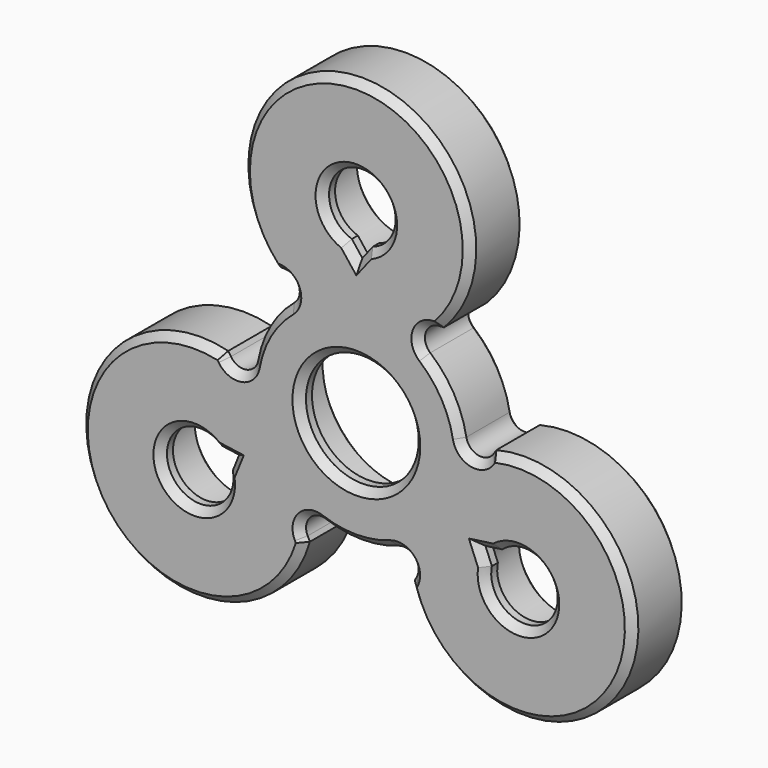
from build123d import *

# Parameters (mm, degrees)
F0_R        = 6.5
F0_R_2      = 11.05
F1_DEPTH    = 9.2
F2_R        = 7.5
F2_R_2      = 4.4268339864
F2_R_3      = 11.05
F3_DEPTH    = 2
F4_R        = 2
F6_DEPTH    = 25
F7_SIZE     = 1
F8_C1_SIZE  = 1
F8_C2_SIZE  = 1
F8_C3_SIZE  = 1
F8_C4_SIZE  = 1
F8_C5_SIZE  = 1
F8_C6_SIZE  = 1
F8_C7_SIZE  = 1
F8_C8_SIZE  = 1
F8_C9_SIZE  = 1
F8_C10_SIZE = 1
F8_C11_SIZE = 1
F8_C12_SIZE = 1
F8_C13_SIZE = 1
F8_C14_SIZE = 1
F8_C15_SIZE = 1
F8_C16_SIZE = 1


with BuildPart() as f1:
    # F0 (on Front) → F1 (new body)
    with BuildSketch(Plane.XZ):
        with BuildLine():
            Line((-10.8594483096, 14.3268800737), (-2.4829795671, 13.8288579597))
            ThreePointArc((-2.4829795671, 13.8288579597), (-12.1676569232, 7.025), (-13.217632082, -4.7641055977))
            Line((-13.217632082, -4.7641055977), (-17.8371662556, 2.2411180703))
            ThreePointArc((-17.8371662556, 2.2411180703), (-34.6870755728, -20.0265924193), (-6.977717946, -16.5679981441))
            Line((-6.977717946, -16.5679981441), (-10.7346525149, -9.064752362))
            ThreePointArc((-10.7346525149, -9.064752362), (0, -14.05), (10.7346525149, -9.064752362))
            Line((10.7346525149, -9.064752362), (6.977717946, -16.5679981441))
            ThreePointArc((6.977717946, -16.5679981441), (34.6870755728, -20.0265924193), (17.8371662556, 2.2411180703))
            Line((17.8371662556, 2.2411180703), (13.217632082, -4.7641055977))
            ThreePointArc((13.217632082, -4.7641055977), (12.1676569232, 7.025), (2.4829795671, 13.8288579597))
            Line((2.4829795671, 13.8288579597), (10.8594483096, 14.3268800737))
            ThreePointArc((10.8594483096, 14.3268800737), (0, 40.0531848387), (-10.8594483096, 14.3268800737))
        make_face()
        with Locations((-21.5623582929, -12.4490333648)):
            Circle(F0_R, mode=Mode.SUBTRACT)
        with Locations((21.5623582929, -12.4490333648)):
            Circle(F0_R, mode=Mode.SUBTRACT)
        Circle(F0_R_2, mode=Mode.SUBTRACT)
        with Locations((0, 24.8980667296)):
            Circle(F0_R, mode=Mode.SUBTRACT)
    extrude(amount=F1_DEPTH)

    # F2 (on face) → F3 (join)
    with BuildSketch(Plane.XZ.offset(9.2)):
        with Locations((0, 24.8980667296)):
            Circle(F2_R)
        with Locations((0, 24.8980667296)):
            Circle(F2_R_2, mode=Mode.SUBTRACT)
        with Locations((-21.5623582929, -12.4490333648)):
            Circle(F2_R)
        with Locations((-21.5623582929, -12.4490333648)):
            Circle(F2_R_2, mode=Mode.SUBTRACT)
        with Locations((21.5623582929, -12.4490333648)):
            Circle(F2_R)
        with Locations((21.5623582929, -12.4490333648)):
            Circle(F2_R_2, mode=Mode.SUBTRACT)
        Circle(F2_R_3)
        Circle(F2_R, mode=Mode.SUBTRACT)
    extrude(amount=-F3_DEPTH)

    # F4
    f4_edges = [f1.edges().sort_by_distance(p)[0] for p in [
        (2.48298, -4.6, 13.828858),
        (-2.48298, -4.6, 13.828858),
        (-13.217632, -4.6, -4.764106),
        (-10.734653, -4.6, -9.064752),
        (10.734653, -4.6, -9.064752),
        (13.217632, -4.6, -4.764106),
    ]]
    fillet(f4_edges, radius=F4_R)

    # F5 (on face) → F6 (cut)
    with BuildSketch(Plane.XZ.offset(9.2)):
        with BuildLine():
            Line((0, 18.9108662307), (1.7659365324, 21.1738422452))
            ThreePointArc((1.7659365324, 21.1738422452), (0, 24.9152206672), (-1.7659365324, 21.1738422452))
            Line((-1.7659365324, 21.1738422452), (0, 18.9108662307))
        make_face()
        with BuildLine():
            Line((-16.3772905634, -9.4554331154), (-19.2200535463, -9.057575224))
            ThreePointArc((-19.2200535463, -9.057575224), (-21.5772140387, -12.4576103336), (-17.4541170138, -12.1162670212))
            Line((-17.4541170138, -12.1162670212), (-16.3772905634, -9.4554331154))
        make_face()
        with BuildLine():
            Line((16.3772905634, -9.4554331154), (17.4541170138, -12.1162670212))
            ThreePointArc((17.4541170138, -12.1162670212), (21.5772140387, -12.4576103336), (19.2200535463, -9.057575224))
            Line((19.2200535463, -9.057575224), (16.3772905634, -9.4554331154))
        make_face()
    extrude(amount=-F6_DEPTH, mode=Mode.SUBTRACT)

    # F7
    f7_edges = [f1.edges().sort_by_distance(p)[0] for p in [
        (10.530932, 0, 14.307348),
        (8.422362, 0, 12.919623),
        (0, 0, 40.053185),
        (12.167657, 0, 7.025),
        (-10.530932, 0, 14.307348),
        (15.399903, 0, 0.834168),
        (-8.422362, 0, 12.919623),
        (17.655993, 0, 1.96638),
        (-12.167657, 0, 7.025),
        (34.687076, 0, -20.026592),
        (-15.399903, 0, 0.834168),
        (7.125061, 0, -16.273728),
        (-17.655993, 0, 1.96638),
        (6.977541, 0, -13.753791),
        (-34.687076, 0, -20.026592),
        (0, 0, -14.05),
        (-7.125061, 0, -16.273728),
        (-6.977541, 0, -13.753791),
        (-28.062358, 0, -12.449033),
        (15.062358, 0, -12.449033),
        (-11.05, 0, 0),
        (-6.5, 0, 24.898067),
    ]]
    chamfer(f7_edges, length=F7_SIZE)

    # F8: chamfer of 1 on 28 edges, made by hand

    # F8_c1
    f8_c1_edges = [f1.edges().sort_by_distance(p)[0] for p in [
        (10.5309316289, -9.2, 14.3073481472),
        (8.4223621743, -9.2, 12.9196228952),
        (17.6559927707, -9.2, 1.9663802425),
        (15.3999027217, -9.2, 0.8341681552),
        (12.1676569232, -9.2, 7.025),
    ]]
    chamfer(f8_c1_edges, length=F8_C1_SIZE)

    # F8_c2
    f8_c2_edges = [f1.edges().sort_by_distance(p)[0] for p in [
        (-10.5309316289, -9.2, 14.3073481472),
        (-8.4223621743, -9.2, 12.9196228952),
        (-12.1676569232, -9.2, 7.025),
        (-15.3999027217, -9.2, 0.8341681552),
        (-17.6559927707, -9.2, 1.9663802425),
    ]]
    chamfer(f8_c2_edges, length=F8_C2_SIZE)

    # F8_c3
    f8_c3_edges = [f1.edges().sort_by_distance(p)[0] for p in [
        (-7.1250611419, -9.2, -16.2737283897),
        (-6.9775405475, -9.2, -13.7537910504),
        (0, -9.2, -14.05),
        (6.9775405475, -9.2, -13.7537910504),
        (7.1250611419, -9.2, -16.2737283897),
    ]]
    chamfer(f8_c3_edges, length=F8_C3_SIZE)

    # F8_c4
    f8_c4_edges = [f1.edges().sort_by_distance(p)[0] for p in [
        (34.6870755728, -9.2, -20.0265924193),
    ]]
    chamfer(f8_c4_edges, length=F8_C4_SIZE)

    # F8_c5
    f8_c5_edges = [f1.edges().sort_by_distance(p)[0] for p in [
        (-25.3961089835, -9.2, -14.662450358),
    ]]
    chamfer(f8_c5_edges, length=F8_C5_SIZE)

    # F8_c6
    f8_c6_edges = [f1.edges().sort_by_distance(p)[0] for p in [
        (-16.7411021229, -9.2, -9.4045159968),
    ]]
    chamfer(f8_c6_edges, length=F8_C6_SIZE)

    # F8_c7
    f8_c7_edges = [f1.edges().sort_by_distance(p)[0] for p in [
        (-16.515100825, -9.2, -9.7959617274),
    ]]
    chamfer(f8_c7_edges, length=F8_C7_SIZE)

    # F8_c8
    f8_c8_edges = [f1.edges().sort_by_distance(p)[0] for p in [
        (25.3961089835, -9.2, -14.662450358),
    ]]
    chamfer(f8_c8_edges, length=F8_C8_SIZE)

    # F8_c9
    f8_c9_edges = [f1.edges().sort_by_distance(p)[0] for p in [
        (16.515100825, -9.2, -9.7959617274),
    ]]
    chamfer(f8_c9_edges, length=F8_C9_SIZE)

    # F8_c10
    f8_c10_edges = [f1.edges().sort_by_distance(p)[0] for p in [
        (16.7411021229, -9.2, -9.4045159968),
    ]]
    chamfer(f8_c10_edges, length=F8_C10_SIZE)

    # F8_c11
    f8_c11_edges = [f1.edges().sort_by_distance(p)[0] for p in [
        (-7.5, -9.2, 0),
    ]]
    chamfer(f8_c11_edges, length=F8_C11_SIZE)

    # F8_c12
    f8_c12_edges = [f1.edges().sort_by_distance(p)[0] for p in [
        (0, -9.2, 29.324900716),
    ]]
    chamfer(f8_c12_edges, length=F8_C12_SIZE)

    # F8_c13
    f8_c13_edges = [f1.edges().sort_by_distance(p)[0] for p in [
        (0.226001298, -9.2, 19.2004777242),
    ]]
    chamfer(f8_c13_edges, length=F8_C13_SIZE)

    # F8_c14
    f8_c14_edges = [f1.edges().sort_by_distance(p)[0] for p in [
        (-0.226001298, -9.2, 19.2004777242),
    ]]
    chamfer(f8_c14_edges, length=F8_C14_SIZE)

    # F8_c15
    f8_c15_edges = [f1.edges().sort_by_distance(p)[0] for p in [
        (0, -9.2, 40.0531848387),
    ]]
    chamfer(f8_c15_edges, length=F8_C15_SIZE)

    # F8_c16
    f8_c16_edges = [f1.edges().sort_by_distance(p)[0] for p in [
        (-34.6870755728, -9.2, -20.0265924193),
    ]]
    chamfer(f8_c16_edges, length=F8_C16_SIZE)


solid = f1.part
